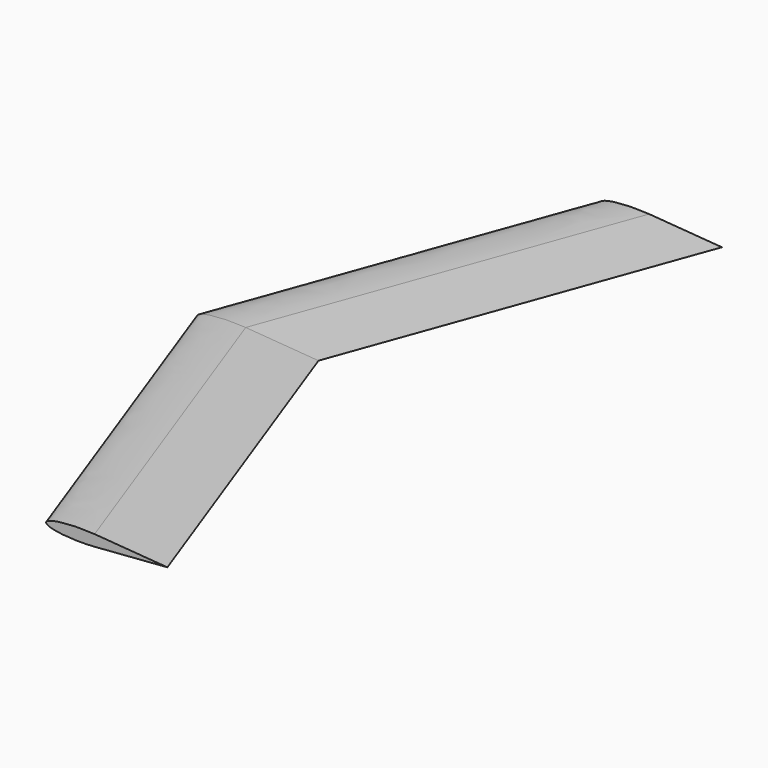
from build123d import *


# Not quite as in the source:
# - a pattern or mirror of a feature is missing from the dataset's text; its kind, count and spacing are read off the source's solid


with BuildPart() as f2:
    # F2: sweep along a path in F1
    with BuildLine(Plane.XY) as f2_path:
        Line((0, 0), (184.8968790072, 508))
    # F0 (on Front) → F2 (sweep)
    with BuildSketch(Plane.XZ):
        with BuildLine():
            add(Edge.make_bspline(
                [(71.12, 8.1478195856), (0, 13.5796993094), (0, 0)],
                knots=[4.3008721343, 4.3008721343, 4.3008721343, 6.2831853072, 6.2831853072, 6.2831853072], degree=2, weights=[1, 0.5477225575, 1]))
            add(Edge.make_bspline(
                [(0, 0), (0, -13.5796993094), (71.12, -8.1478195856)],
                knots=[0, 0, 0, 1.9823131729, 1.9823131729, 1.9823131729], degree=2, weights=[1, 0.5477225575, 1]))
            add(Edge.make_bspline(
                [(71.12, -8.1478195856), (177.8, 0), (71.12, 8.1478195856)],
                knots=[1.9823131729, 1.9823131729, 1.9823131729, 4.3008721343, 4.3008721343, 4.3008721343], degree=2, weights=[1, 0.4, 1]))
        make_face()
        with BuildLine():
            add(Edge.make_bspline(
                [(71.12, -8.1478195856), (177.8, 0), (71.12, 8.1478195856)],
                knots=[1.9823131729, 1.9823131729, 1.9823131729, 4.3008721343, 4.3008721343, 4.3008721343], degree=2, weights=[1, 0.4, 1]))
            Line((71.12, -8.1478195856), (177.8, 0))
            Line((177.8, 0), (71.12, 8.1478195856))
        make_face()
    sweep(path=f2_path.line)

    # F2_copies: F2 across plane


with BuildPart() as f2_1:
    add(f2.part)
    add(f2.part.mirror(Plane(origin=(0, 0, 0), x_dir=(0, 0, -1), z_dir=(0, -1, 0))))


solid = f2_1.part
